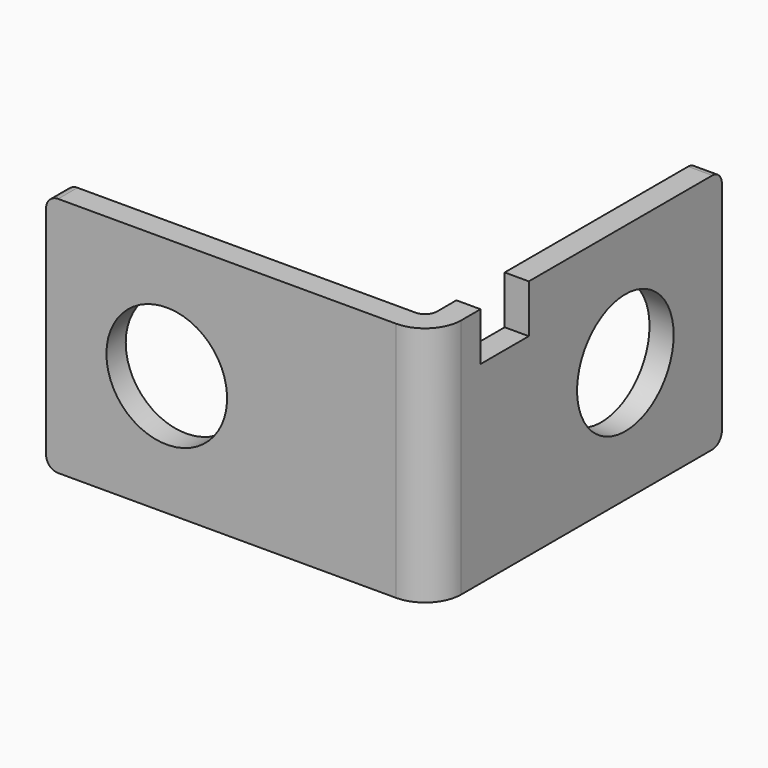
from build123d import *

# Parameters (mm, degrees)
F0_W     = 2
F0_H     = 20
F1_DEPTH = 30
F2_R     = 5
F3_DEPTH = 2
F4_R     = 5
F5_DEPTH = 2
F6_R     = 1
F7_R     = 3


with BuildPart() as f1:
    # F0 (on Right) → F1 (new body)
    with BuildSketch(Plane.YZ):
        with Locations((1, 10)):
            Rectangle(F0_W, F0_H)
    extrude(amount=F1_DEPTH)

    # F2 (on face) → F3 (cut)
    with BuildSketch(Plane(origin=(0, 2, 0), x_dir=(-1, 0, 0), z_dir=(0, 1, 0))):
        with Locations((-10, 10)):
            Circle(F2_R)
    extrude(amount=-F3_DEPTH, mode=Mode.SUBTRACT)

    # F4 (on face) → F5 (join)
    with BuildSketch(Plane.YZ.offset(30)):
        Polygon((0, 20), (0, 0), (30, 0), (30, 20), (10, 20), (10, 16), (5, 16), (5, 20), align=None)
        with Locations((20, 10)):
            Circle(F4_R, mode=Mode.SUBTRACT)
    extrude(amount=F5_DEPTH)

    # F6
    f6_edges = [f1.edges().sort_by_distance(p)[0] for p in [
        (30, 2, 10),
        (31, 30, 0),
        (0, 1, 20),
        (0, 1, 0),
        (31, 30, 20),
    ]]
    fillet(f6_edges, radius=F6_R)

    # F7
    f7_edges = [f1.edges().sort_by_distance(p)[0] for p in [
        (32, 0, 10),
    ]]
    fillet(f7_edges, radius=F7_R)


solid = f1.part
